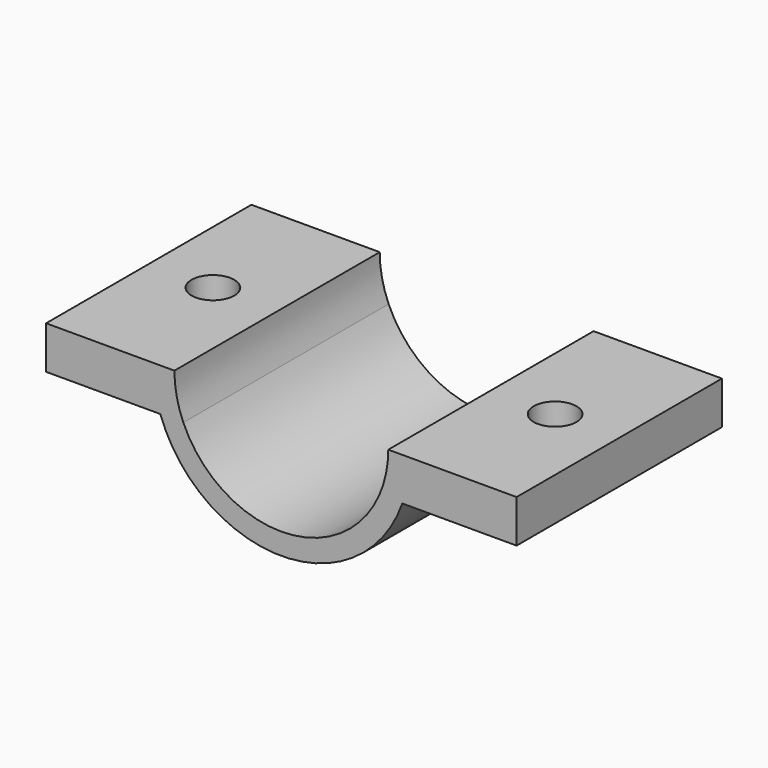
from build123d import *

# Parameters (mm, degrees)
F1_DEPTH = 30
F3_D     = 5


with BuildPart() as f1:
    # F0 (on Front) → F1 (new body)
    with BuildSketch(Plane.XZ):
        with BuildLine():
            ThreePointArc((-14.1421356237, -5), (-14.7839783948, -2.5365296809), (-15, 0))
            Line((-15, 0), (-27.5, 0))
            Line((-27.5, 0), (-27.5, -5))
            Line((-27.5, -5), (-14.1421356237, -5))
        make_face()
        with BuildLine():
            ThreePointArc((-11.4564392374, -5), (-12.2363289116, -2.5538705461), (-12.5, 0))
            Line((-12.5, 0), (-15, 0))
            ThreePointArc((-15, 0), (-14.7839783948, -2.5365296809), (-14.1421356237, -5))
            Line((-14.1421356237, -5), (-11.4564392374, -5))
        make_face()
        with BuildLine():
            ThreePointArc((11.4564392374, -5), (0, -12.5), (-11.4564392374, -5))
            Line((-11.4564392374, -5), (-14.1421356237, -5))
            ThreePointArc((-14.1421356237, -5), (0, -15), (14.1421356237, -5))
            Line((14.1421356237, -5), (11.4564392374, -5))
        make_face()
        with BuildLine():
            ThreePointArc((12.5, 0), (12.2363289116, -2.5538705461), (11.4564392374, -5))
            Line((11.4564392374, -5), (14.1421356237, -5))
            ThreePointArc((14.1421356237, -5), (14.7839783948, -2.5365296809), (15, 0))
            Line((15, 0), (12.5, 0))
        make_face()
        with BuildLine():
            ThreePointArc((15, 0), (14.7839783948, -2.5365296809), (14.1421356237, -5))
            Line((14.1421356237, -5), (27.5, -5))
            Line((27.5, -5), (27.5, 0))
            Line((27.5, 0), (15, 0))
        make_face()
    extrude(amount=F1_DEPTH)

    # F3 (through all)
    with Locations(Plane.XY):
        with Locations((-20, -15), (20, -15)):
            Hole(F3_D / 2)


solid = f1.part
